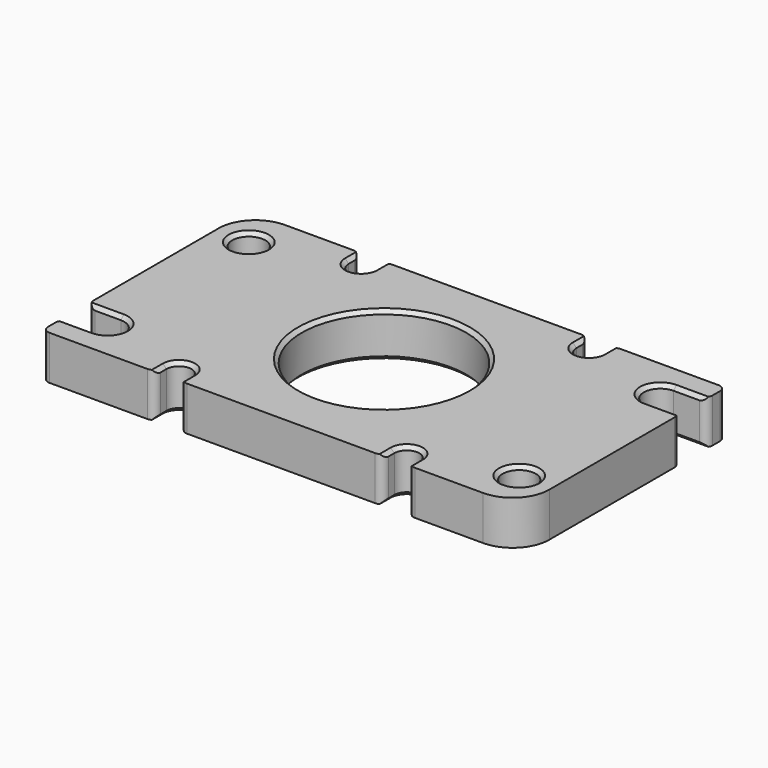
from build123d import *

# Parameters (mm, degrees)
F0_R     = 2.25
F0_R_2   = 11.2
F1_DEPTH = 6
F2_SIZE  = 0.5
F3_R     = 1


with BuildPart() as f1:
    # F0 (on Top) → F1 (new body)
    with BuildSketch(Plane.XY):
        with BuildLine():
            Line((-17.2, 17.5), (-27.5, 17.5))
            ThreePointArc((-27.5, 17.5), (-31.0355339059, 16.0355339059), (-32.5, 12.5))
            Line((-32.5, 12.5), (-32.5, -9.75))
            Line((-32.5, -9.75), (-28, -9.75))
            ThreePointArc((-28, -9.75), (-26.4090097423, -10.4090097423), (-25.75, -12))
            ThreePointArc((-25.75, -12), (-26.4090097423, -13.5909902577), (-28, -14.25))
            Line((-28, -14.25), (-32.5, -14.25))
            Line((-32.5, -14.25), (-32.5, -17.5))
            Line((-32.5, -17.5), (-17.2, -17.5))
            Line((-17.2, -17.5), (-17.2, -15.5))
            ThreePointArc((-17.2, -15.5), (-15.5, -13.8), (-13.8, -15.5))
            Line((-13.8, -15.5), (-13.8, -17.5))
            Line((-13.8, -17.5), (13.8, -17.5))
            Line((13.8, -17.5), (13.8, -15.5))
            ThreePointArc((13.8, -15.5), (15.5, -13.8), (17.2, -15.5))
            Line((17.2, -15.5), (17.2, -17.5))
            Line((17.2, -17.5), (27.5, -17.5))
            ThreePointArc((27.5, -17.5), (31.0355339059, -16.0355339059), (32.5, -12.5))
            Line((32.5, -12.5), (32.5, 9.75))
            Line((32.5, 9.75), (28, 9.75))
            ThreePointArc((28, 9.75), (25.75, 12), (28, 14.25))
            Line((28, 14.25), (32.5, 14.25))
            Line((32.5, 14.25), (32.5, 17.5))
            Line((32.5, 17.5), (17.2, 17.5))
            Line((17.2, 17.5), (17.2, 15.5))
            ThreePointArc((17.2, 15.5), (15.5, 13.8), (13.8, 15.5))
            Line((13.8, 15.5), (13.8, 17.5))
            Line((13.8, 17.5), (-13.8, 17.5))
            Line((-13.8, 17.5), (-13.8, 15.5))
            ThreePointArc((-13.8, 15.5), (-15.5, 13.8), (-17.2, 15.5))
            Line((-17.2, 15.5), (-17.2, 17.5))
        make_face()
        with Locations((28, -12)):
            Circle(F0_R, mode=Mode.SUBTRACT)
        with Locations((-28, 12)):
            Circle(F0_R, mode=Mode.SUBTRACT)
        Circle(F0_R_2, mode=Mode.SUBTRACT)
    extrude(amount=F1_DEPTH)

    # F2
    f2_edges = [f1.edges().sort_by_distance(p)[0] for p in [
        (-11.2, 0, 6),
        (-11.2, 0, 0),
        (-25.75, -12, 0),
        (-15.5, -13.8, 0),
        (15.5, -13.8, 0),
        (25.75, -12, 0),
        (25.75, 12, 0),
        (15.5, 13.8, 0),
        (-15.5, 13.8, 0),
        (-30.25, 12, 0),
        (-30.25, 12, 6),
        (-15.5, 13.8, 6),
        (15.5, 13.8, 6),
        (25.75, 12, 6),
        (-25.75, -12, 6),
        (-15.5, -13.8, 6),
        (15.5, -13.8, 6),
        (25.75, -12, 6),
        (-13.8, 16.5, 6),
        (-17.2, 16.5, 6),
        (-30.25, -9.75, 6),
        (-30.25, -14.25, 6),
        (-17.2, -16.5, 6),
        (-13.8, -16.5, 6),
        (13.8, -16.5, 6),
        (17.2, -16.5, 6),
        (30.25, 9.75, 6),
        (30.25, 14.25, 6),
        (17.2, 16.5, 6),
        (13.8, 16.5, 6),
        (17.2, 16.5, 0),
        (30.25, 14.25, 0),
        (30.25, 9.75, 0),
        (17.2, -16.5, 0),
        (13.8, -16.5, 0),
        (-13.8, -16.5, 0),
        (-17.2, -16.5, 0),
        (-30.25, -14.25, 0),
        (-30.25, -9.75, 0),
        (-17.2, 16.5, 0),
        (-13.8, 16.5, 0),
        (13.8, 16.5, 0),
    ]]
    chamfer(f2_edges, length=F2_SIZE)

    # F3
    f3_edges = [f1.edges().sort_by_distance(p)[0] for p in [
        (-32.5, -14.25, 3),
        (-32.5, -9.75, 3),
        (-32.5, -17.5, 3),
        (-17.2, -17.5, 3),
        (-13.8, -17.5, 3),
        (13.8, -17.5, 3),
        (17.2, -17.5, 3),
        (32.5, 14.25, 3),
        (32.5, 9.75, 3),
        (32.5, 17.5, 3),
        (17.2, 17.5, 3),
        (13.8, 17.5, 3),
        (-13.8, 17.5, 3),
        (-17.2, 17.5, 3),
    ]]
    fillet(f3_edges, radius=F3_R)


solid = f1.part
